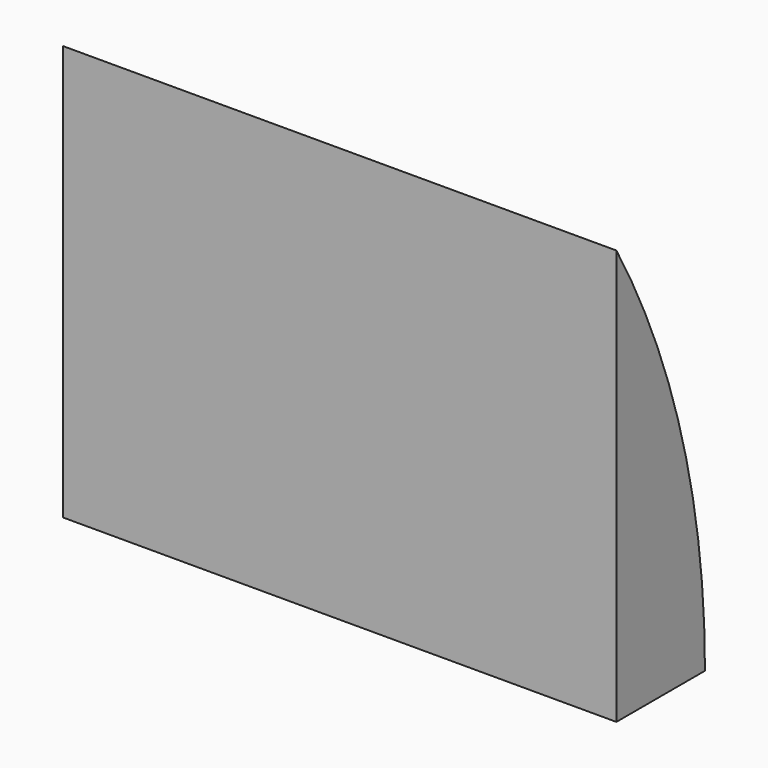
from build123d import *

# Parameters (mm, degrees)
F0_W        = 20
F0_H        = 15
F1_DEPTH    = 4
F2_T1_DEPTH = 94.8331477355


# Not quite as in the source:
# - a fillet or chamfer that OpenCascade refuses, or shapes differently, is made with other operations: its cross-section is extruded or revolved along the edge and cut away or added


with BuildPart() as f1:
    # F0 (on Front) → F1 (new body)
    with BuildSketch(Plane.XZ):
        with Locations((10, 7.5)):
            Rectangle(F0_W, F0_H)
    extrude(amount=F1_DEPTH)

    # F2: fillet of radius 30 on 1 edges, made by hand

    # F2_s2 → F2_t1 (cut)
    with BuildSketch(Plane.YZ.offset(-37.4165738677)):
        with BuildLine():
            ThreePointArc((-4, 15), (-1.0172465076, 7.7793371453), (0, 0.0333704529))
            Line((0, 0.0333704529), (0.6, 0.0333704529))
            Line((0.6, 0.0333704529), (0.6, 15))
            Line((0.6, 15), (0, 15.6))
            ThreePointArc((0, 15.6), (-2, 15.6), (-3.48, 15.2993325909))
            Line((-3.48, 15.2993325909), (-4, 15))
        make_face()
    extrude(amount=F2_T1_DEPTH, mode=Mode.SUBTRACT)


solid = f1.part
